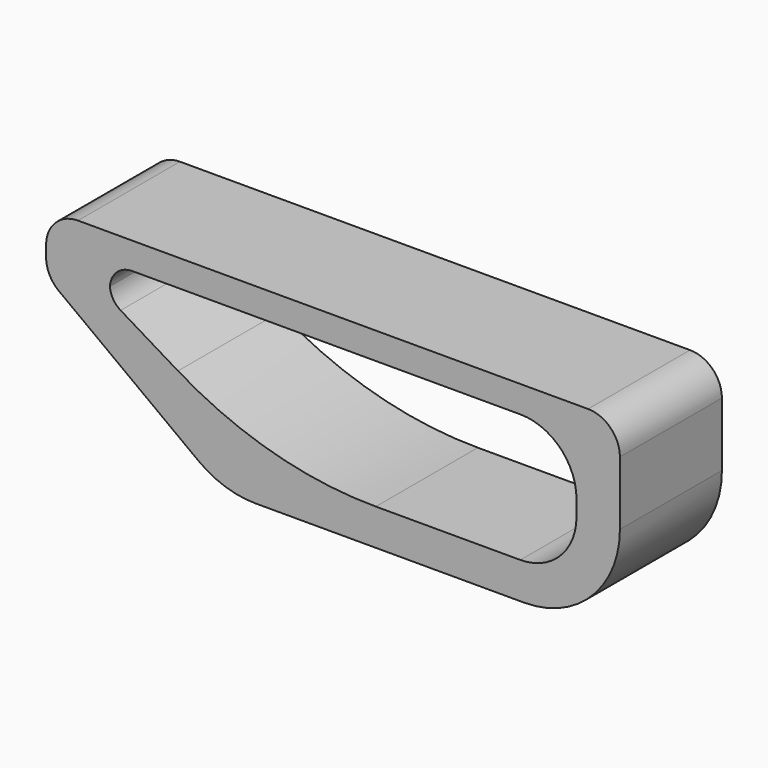
from build123d import *

# Parameters (mm, degrees)
F1_DEPTH    = 101.6
F2_R        = 25.4
F3_R        = 76.2
F4_R        = 25.4
F5_T1_DEPTH = 101.6
F6_R        = 44.7643478735
F7_R        = 304.8


# Not quite as in the source:
# - a fillet or chamfer that OpenCascade refuses, or shapes differently, is made with other operations: its cross-section is extruded or revolved along the edge and cut away or added


with BuildPart() as f1:
    # F0 (on Front) → F1 (new body)
    with BuildSketch(Plane.XZ):
        Polygon((228.6, -76.2), (228.6, 76.2), (-228.6, 76.2), (-228.6, 29.4590149546), (-86.9704671455, -76.2), align=None)
        Polygon((-50.8129218496, -47.2383520842), (-177.8, 29.4590149546), (-177.8, 54.8590149546), (194.0227749825, 54.8590149546), (194.0227749825, -47.2383520842), align=None, mode=Mode.SUBTRACT)
    extrude(amount=F1_DEPTH)

    # F2
    f2_edges = [f1.edges().sort_by_distance(p)[0] for p in [
        (-228.6, -50.8, 76.2),
        (-228.6, -50.8, 29.459015),
    ]]
    fillet(f2_edges, radius=F2_R)

    # F3
    f3_edges = [f1.edges().sort_by_distance(p)[0] for p in [
        (-86.970467, -50.8, -76.2),
        (228.6, -50.8, -76.2),
    ]]
    fillet(f3_edges, radius=F3_R)

    # F4
    f4_edges = [f1.edges().sort_by_distance(p)[0] for p in [
        (228.6, -50.8, 76.2),
    ]]
    fillet(f4_edges, radius=F4_R)

    # F5: fillet of radius 17.78 on 2 edges, made by hand

    # F5_s2 → F5_t1 (join)
    with BuildSketch(Plane.XZ):
        with BuildLine():
            ThreePointArc((-169.2122093999, 24.2721806932), (-175.5049262693, 30.7540427919), (-177.8, 39.4916316146))
            Line((-177.8, 39.4916316146), (-177.8, 29.4590149546))
            Line((-177.8, 29.4590149546), (-169.2122093999, 24.2721806932))
        make_face()
        with BuildLine():
            ThreePointArc((-177.8, 37.0790149546), (-172.5923585695, 49.6513735241), (-160.02, 54.8590149546))
            Line((-160.02, 54.8590149546), (-177.8, 54.8590149546))
            Line((-177.8, 54.8590149546), (-177.8, 37.0790149546))
        make_face()
    extrude(amount=F5_T1_DEPTH)

    # F6
    f6_edges = [f1.edges().sort_by_distance(p)[0] for p in [
        (194.022775, -50.8, -47.238352),
        (194.022775, -50.8, 54.859015),
    ]]
    fillet(f6_edges, radius=F6_R)

    # F7
    f7_edges = [f1.edges().sort_by_distance(p)[0] for p in [
        (-50.812922, -50.8, -47.238352),
    ]]
    fillet(f7_edges, radius=F7_R)


solid = f1.part
